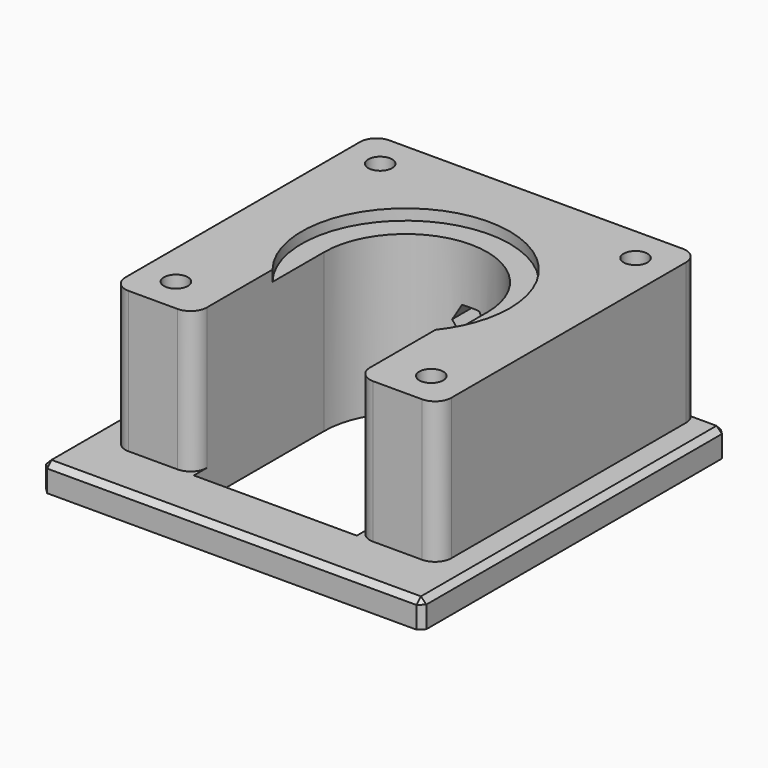
from build123d import *

# Parameters (mm, degrees)
F0_W      = 70
F0_H      = 70
F1_DEPTH  = 5
F2_W      = 60
F2_H      = 60
F3_DEPTH  = 26
F4_R      = 2.2
F5_DEPTH  = 10
F6_DEPTH  = 31.001
F7_DEPTH  = 2
F8_R      = 1.6
F9_DEPTH  = 70.001
F10_START = -7
F10_DEPTH = 18
F11_R     = 3
F12_SIZE  = 1


with BuildPart() as f1:
    # F0 (on Top) → F1 (new body)
    with BuildSketch(Plane.XY):
        Rectangle(F0_W, F0_H)
    extrude(amount=F1_DEPTH)

    # F2 (on face) → F3 (join)
    with BuildSketch(Plane.XY.offset(5)):
        with Locations((0, 5)):
            Rectangle(F2_W, F2_H)
    extrude(amount=F3_DEPTH)

    # F4 (on face) → F5 (cut)
    with BuildSketch(Plane.XY.offset(31)):
        with Locations((-23.5, -18.5)):
            Circle(F4_R)
        with Locations((-23.5, 28.5)):
            Circle(F4_R)
        with Locations((23.5, 28.5)):
            Circle(F4_R)
        with Locations((23.5, -18.5)):
            Circle(F4_R)
    extrude(amount=-F5_DEPTH, mode=Mode.SUBTRACT)

    # F4 (on face) → F6 (cut, through all)
    with BuildSketch(Plane.XY.offset(31)):
        with BuildLine():
            ThreePointArc((-15, 5), (0, -10), (15, 5))
            ThreePointArc((15, 5), (0, 20), (-15, 5))
        make_face()
        with BuildLine():
            Line((15, -6.9047259523), (15, 5))
            ThreePointArc((15, 5), (0, -10), (-15, 5))
            Line((-15, 5), (-15, -6.9047259523))
            ThreePointArc((-15, -6.9047259523), (0, -14.15), (15, -6.9047259523))
        make_face()
        with BuildLine():
            Line((15, -25), (15, -6.9047259523))
            ThreePointArc((15, -6.9047259523), (0, -14.15), (-15, -6.9047259523))
            Line((-15, -6.9047259523), (-15, -25))
            Line((-15, -25), (15, -25))
        make_face()
    extrude(amount=-F6_DEPTH, mode=Mode.SUBTRACT)

    # F4 (on face) → F7 (cut)
    with BuildSketch(Plane.XY.offset(31)):
        with BuildLine():
            ThreePointArc((-15, 5), (0, 20), (15, 5))
            Line((15, 5), (15, -6.9047259523))
            ThreePointArc((15, -6.9047259523), (18.0827611277, -1.3036695662), (19.15, 5))
            ThreePointArc((19.15, 5), (-6.3036695662, 23.0827611277), (-15, -6.9047259523))
            Line((-15, -6.9047259523), (-15, 5))
        make_face()
    extrude(amount=-F7_DEPTH, mode=Mode.SUBTRACT)

    # F8 (on face) → F9 (cut, through all)
    with BuildSketch(Plane(origin=(0, 35, 0), x_dir=(-1, 0, 0), z_dir=(0, 1, 0))):
        with Locations((0, 16)):
            Circle(F8_R)
    extrude(amount=-F9_DEPTH, mode=Mode.SUBTRACT)

    # F8 (on face) → F10 (cut)
    with BuildSketch(Plane(origin=(0, 35, 0), x_dir=(-1, 0, 0), z_dir=(0, 1, 0)).offset(F10_START)):
        Polygon((3.1754264805, 16), (1.5877132403, 18.75), (-1.5877132403, 18.75), (-3.1754264805, 16), (-1.5877132403, 13.25), (1.5877132403, 13.25), align=None)
        with Locations((0, 16)):
            Circle(F8_R, mode=Mode.SUBTRACT)
    extrude(amount=-F10_DEPTH, mode=Mode.SUBTRACT)

    # F11
    f11_edges = [f1.edges().sort_by_distance(p)[0] for p in [
        (30, -25, 18),
        (-30, -25, 18),
        (30, 35, 18),
        (-30, 35, 18),
        (-15, -25, 18),
        (15, -25, 18),
    ]]
    fillet(f11_edges, radius=F11_R)

    # F12
    f12_edges = [f1.edges().sort_by_distance(p)[0] for p in [
        (-35, 0, 5),
        (0, -35, 5),
        (35, 0, 5),
        (32.5, 35, 5),
        (-32.5, 35, 5),
        (35, -35, 2.5),
        (-35, -35, 2.5),
        (-35, 35, 2.5),
        (35, 35, 2.5),
    ]]
    chamfer(f12_edges, length=F12_SIZE)


solid = f1.part
